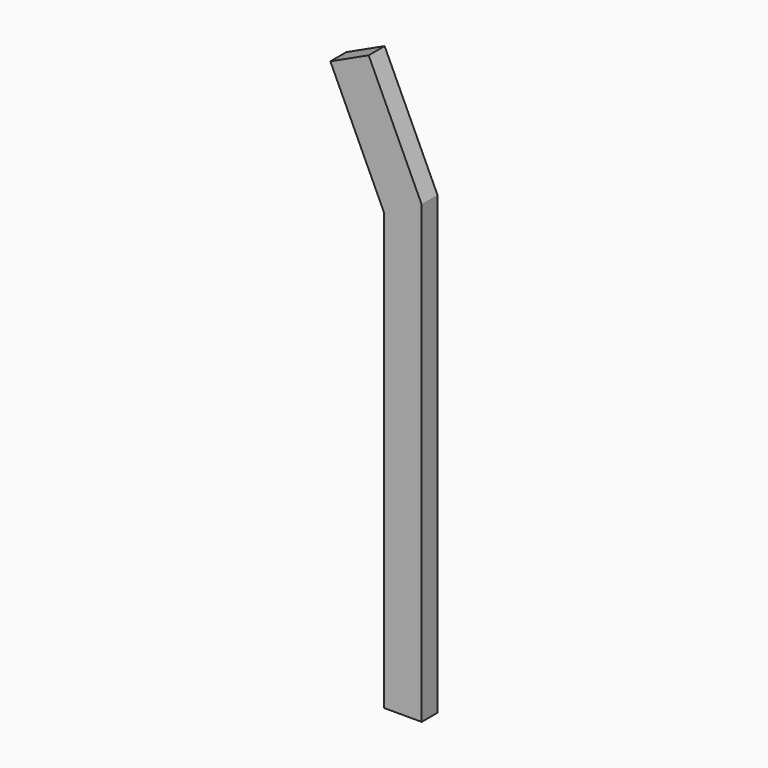
from build123d import *

# Parameters (mm, degrees)
F1_DEPTH = 38.1


with BuildPart() as f1:
    # F0 (on Front) → F1 (new body)
    with BuildSketch(Plane.XZ):
        Polygon((118.6708062887, 832.2721719742), (118.6708062887, 0), (190.5, 0), (190.5, 869.0049764808), (89.367787617, 1087.0554128251), (16.2338521332, 1053.1357526779), align=None)
    extrude(amount=-F1_DEPTH)


solid = f1.part
